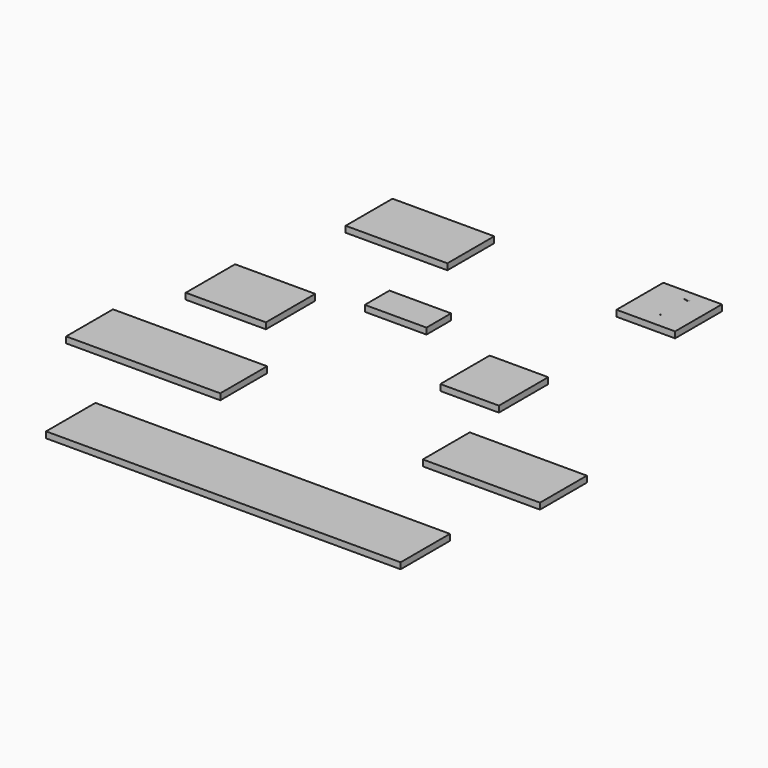
from build123d import *

# Parameters (mm, degrees)
F0_W          = 25.4
F0_H          = 12.7
F1_DEPTH      = 2.54
F2_W          = 24.13
F2_H          = 24.13
F3_DEPTH      = 2.54
F4_W          = 41.91
F4_H          = 24.13
F5_DEPTH      = 2.54
F6_W          = 48.26
F6_H          = 24.13
F7_DEPTH      = 2.54
F8_W          = 63.5
F8_H          = 24.13
F9_DEPTH      = 2.54
F10_W         = 24.13
F10_H         = 25.4
F11_DEPTH     = 2.54
F12_W         = 33.02
F12_H         = 25.4
F13_DEPTH     = 2.54
F14_W         = 146.05
F14_H         = 25.4
F15_DEPTH     = 2.54
F16_TEXT_SIZE = 5.5449445628
F17_DEPTH     = 0.0254


# Not quite as in the source:
# - Text() gives the source's letters only with a copy of the font that has no kerning and outlines rounded to 1/6400 em; it was checked with that copy


with BuildPart() as f1:
    # F0 (on Top) → F1 (new body)
    with BuildSketch(Plane.XY):
        with Locations((-11.3194507912, -6.35)):
            Rectangle(F0_W, F0_H)
    extrude(amount=F1_DEPTH)


with BuildPart() as f3:
    # F2 (on Top) → F3 (new body)
    with BuildSketch(Plane.XY):
        with Locations((53.4110925549, 47.2596173521)):
            Rectangle(F2_W, F2_H)
    extrude(amount=F3_DEPTH)


with BuildPart() as f5:
    # F4 (on Top) → F5 (new body)
    with BuildSketch(Plane.XY):
        with Locations((-42.2987812966, 38.5353583415)):
            Rectangle(F4_W, F4_H)
    extrude(amount=F5_DEPTH)


with BuildPart() as f7:
    # F6 (on Top) → F7 (new body)
    with BuildSketch(Plane.XY):
        with Locations((81.9625673676, -73.0648562312)):
            Rectangle(F6_W, F6_H)
    extrude(amount=F7_DEPTH)


with BuildPart() as f9:
    # F8 (on Top) → F9 (new body)
    with BuildSketch(Plane.XY):
        with Locations((-53.5612823169, -77.8127722442)):
            Rectangle(F8_W, F8_H)
    extrude(amount=F9_DEPTH)


with BuildPart() as f11:
    # F10 (on Top) → F11 (new body)
    with BuildSketch(Plane.XY):
        with Locations((41.4818936861, -27.9021533206)):
            Rectangle(F10_W, F10_H)
    extrude(amount=F11_DEPTH)


with BuildPart() as f13:
    # F12 (on Top) → F13 (new body)
    with BuildSketch(Plane.XY):
        with Locations((-57.7537726026, -29.3946098536)):
            Rectangle(F12_W, F12_H)
    extrude(amount=F13_DEPTH)


with BuildPart() as f15:
    # F14 (on Top) → F15 (new body)
    with BuildSketch(Plane.XY):
        with Locations((24.0096701031, -132.8741163015)):
            Rectangle(F14_W, F14_H)
    extrude(amount=F15_DEPTH)


with BuildPart() as f17:
    # F16 (on face) → F17 (new body)
    with BuildSketch(Plane.XY.offset(2.54)):
        with Locations((53.0021041632, 52.6922792196)):
            Text('~', F16_TEXT_SIZE, font='Open Sans', text_align=(TextAlign.LEFT, TextAlign.BOTTOM))
        with Locations((53.0021041632, 37.6100300087)):
            Text('`', F16_TEXT_SIZE, font='Open Sans', text_align=(TextAlign.LEFT, TextAlign.BOTTOM))
    extrude(amount=F17_DEPTH)


solid = Compound([f1.part, f3.part, f5.part, f7.part, f9.part, f11.part, f13.part, f15.part, f17.part])
